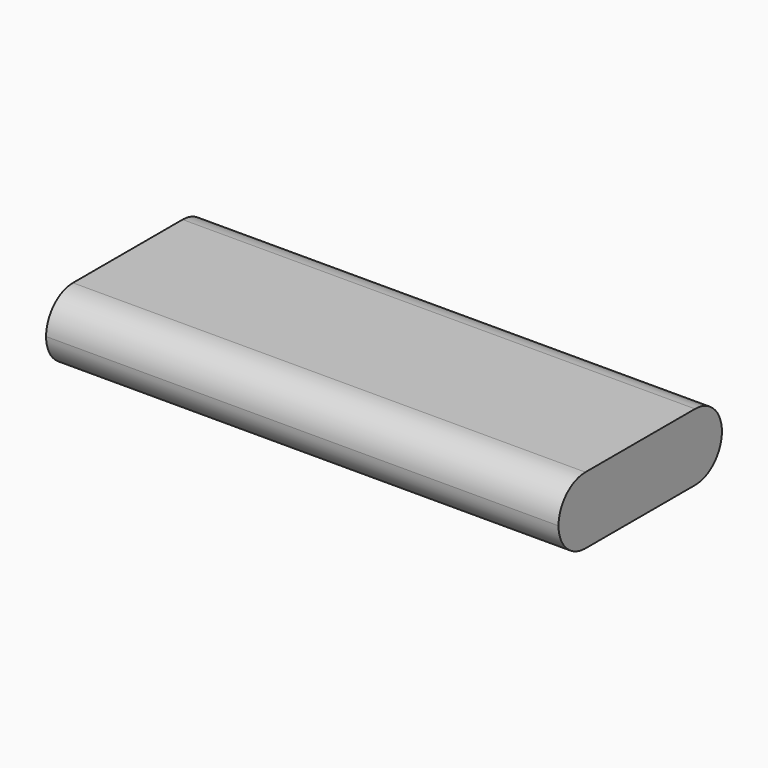
from build123d import *

# Parameters (mm, degrees)
F0_W     = 45.8
F0_H     = 18.25
F1_DEPTH = 6
F2_R     = 2.99999


# Not quite as in the source:
# - a fillet or chamfer is up to 0.001 mm smaller than in the source, because OpenCascade refuses the exact size


with BuildPart() as f1:
    # F0 (on Top) → F1 (new body)
    with BuildSketch(Plane.XY):
        Rectangle(F0_W, F0_H)
    extrude(amount=F1_DEPTH)

    # F2 (radius 3 in the source; OpenCascade refuses exactly that, so slightly less here)
    f2_edges = [f1.edges().sort_by_distance(p)[0] for p in [
        (0, -9.125, 6),
        (0, -9.125, 0),
        (0, 9.125, 6),
        (0, 9.125, 0),
    ]]
    fillet(f2_edges, radius=F2_R)


solid = f1.part
